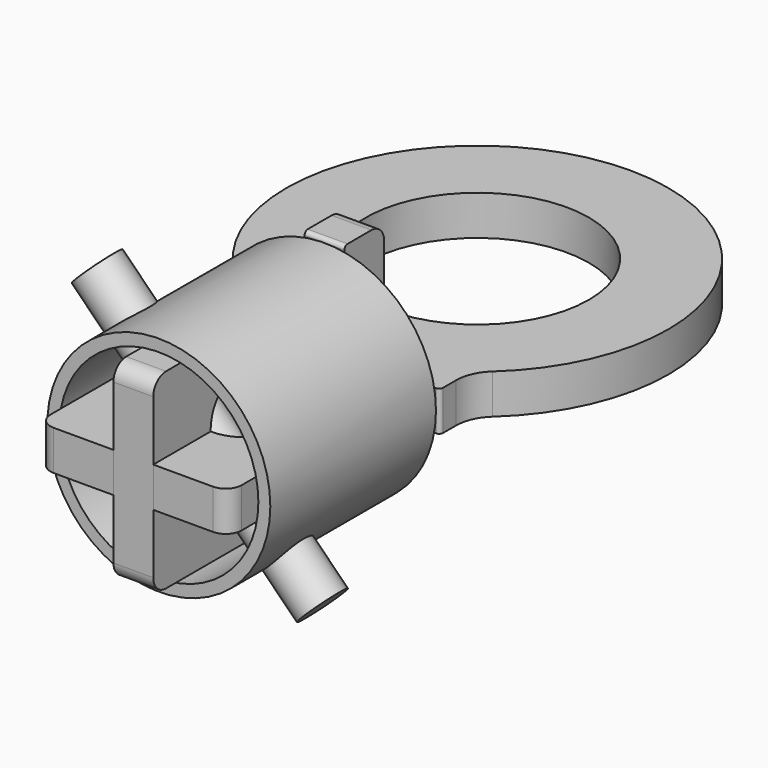
from build123d import *

# Parameters (mm, degrees)
F0_R      = 14
F1_DEPTH  = 2.5
F3_DEPTH  = 2.5
F6_START  = 24
F5_R      = 14
F5_R_2    = 12.5
F6_DEPTH  = 26
F8_R      = 3
F9_DEPTH  = 20
F13_DEPTH = 12.5
F16_DEPTH = 12.5
F17_R     = 2
F17_2_R   = 2
F18_R     = 2
F19_R     = 0.5
F19_2_R   = 0.5


with BuildPart() as f1:
    # F0 (on Top) → F1 (new body, symmetric)
    with BuildSketch(Plane.XY):
        with BuildLine():
            ThreePointArc((14.5, -21.4650879337), (14.9277825496, -19.4415199002), (16.1379310345, -17.7642107037))
            ThreePointArc((16.1379310345, -17.7642107037), (0, 24), (-16.1379310345, -17.7642107037))
            ThreePointArc((-16.1379310345, -17.7642107037), (-14.9277825496, -19.4415199002), (-14.5, -21.4650879337))
            Line((-14.5, -21.4650879337), (-14.5, -24))
            Line((-14.5, -24), (-12, -24))
            Line((-12, -24), (-12, -54))
            Line((-12, -54), (-2.5, -54))
            Line((-2.5, -54), (-2.5, -34))
            Line((-2.5, -34), (2.5, -34))
            Line((2.5, -34), (2.5, -54))
            Line((2.5, -54), (12, -54))
            Line((12, -54), (12, -24))
            Line((12, -24), (14.5, -24))
            Line((14.5, -24), (14.5, -21.4650879337))
        make_face()
        Circle(F0_R, mode=Mode.SUBTRACT)
    extrude(amount=F1_DEPTH, both=True)


with BuildPart() as f3:
    # F2 (on Right) → F3 (new body, symmetric)
    with BuildSketch(Plane.YZ):
        Polygon((-24, 14.5), (-24, 12), (-54, 12), (-54, -12), (-24, -12), (-24, -14.5), (-17.7642107037, -14.5), (-17.7642107037, 14.5), align=None)
    extrude(amount=F3_DEPTH, both=True)

    # F4: cut F1
    add(f1.part, mode=Mode.SUBTRACT)


with BuildPart() as f6:
    # F5 (on Front) → F6 (new body)
    with BuildSketch(Plane.XZ.offset(F6_START)):
        Circle(F5_R)
        Circle(F5_R_2, mode=Mode.SUBTRACT)
    extrude(amount=F6_DEPTH)


with BuildPart() as f9:
    # F8 (on face) → F9 (new body, symmetric)
    with BuildSketch(Plane(origin=(0, 0, 0), x_dir=(0, 1, 0), z_dir=(0.7071067812, 0, -0.7071067812))):
        with Locations((-42, 0)):
            Circle(F8_R)
    extrude(amount=F9_DEPTH, both=True)


with BuildPart() as f6_1:
    add(f6.part)

    # F10: cut F9
    add(f9.part, mode=Mode.SUBTRACT)


with BuildPart() as f3_1:
    add(f3.part)

    # F11: cut F9
    add(f9.part, mode=Mode.SUBTRACT)

    # F15 (on Right) → F16 (cut, symmetric)
    with BuildSketch(Plane.YZ):
        with BuildLine():
            Line((-45, 2.5), (-45, -2.5))
            add(Edge.make_bspline(
                [(-45, -2.5), (-45, -6.7426406871), (-42, -6.7426406871), (-39, -6.7426406871), (-39, -2.5)],
                knots=[1.5707963268, 1.5707963268, 1.5707963268, 3.1415926536, 3.1415926536, 4.7123889804, 4.7123889804, 4.7123889804], degree=2, weights=[1, 0.7071067812, 1, 0.7071067812, 1]))
            Line((-39, -2.5), (-39, 2.5))
            add(Edge.make_bspline(
                [(-39, 2.5), (-39, 6.7426406871), (-42, 6.7426406871), (-45, 6.7426406871), (-45, 2.5)],
                knots=[1.5707963268, 1.5707963268, 1.5707963268, 3.1415926536, 3.1415926536, 4.7123889804, 4.7123889804, 4.7123889804], degree=2, weights=[1, 0.7071067812, 1, 0.7071067812, 1]))
        make_face()
    extrude(amount=F16_DEPTH, both=True, mode=Mode.SUBTRACT)

    # F17#2
    f17_2_edges = [f3_1.edges().sort_by_distance(p)[0] for p in [
        (0, -54, 12),
        (0, -54, -12),
    ]]
    fillet(f17_2_edges, radius=F17_2_R)

    # F18
    f18_edges = [f3_1.edges().sort_by_distance(p)[0] for p in [
        (0, -17.764211, -14.5),
        (0, -17.764211, 14.5),
    ]]
    fillet(f18_edges, radius=F18_R)

    # F19#2
    f19_2_edges = [f3_1.edges().sort_by_distance(p)[0] for p in [
        (0, -24, 14.5),
        (0, -24, -14.5),
    ]]
    fillet(f19_2_edges, radius=F19_2_R)


with BuildPart() as f1_1:
    add(f1.part)

    # F11: cut F9
    add(f9.part, mode=Mode.SUBTRACT)


with BuildPart() as f13:
    # F12 (on Top) → F13 (new body, symmetric)
    with BuildSketch(Plane.XY):
        with BuildLine():
            Line((2.5, -39), (-2.5, -39))
            add(Edge.make_bspline(
                [(-2.5, -39), (-6.7426406871, -39), (-6.7426406871, -42), (-6.7426406871, -45), (-2.5, -45)],
                knots=[4.7123889804, 4.7123889804, 4.7123889804, 6.2831853072, 6.2831853072, 7.853981634, 7.853981634, 7.853981634], degree=2, weights=[1, 0.7071067812, 1, 0.7071067812, 1]))
            Line((-2.5, -45), (2.5, -45))
            add(Edge.make_bspline(
                [(2.5, -45), (6.7426406871, -45), (6.7426406871, -42), (6.7426406871, -39), (2.5, -39)],
                knots=[4.7123889804, 4.7123889804, 4.7123889804, 6.2831853072, 6.2831853072, 7.853981634, 7.853981634, 7.853981634], degree=2, weights=[1, 0.7071067812, 1, 0.7071067812, 1]))
        make_face()
    extrude(amount=F13_DEPTH, both=True)


with BuildPart() as f1_2:
    add(f1_1.part)

    # F14: cut F13
    add(f13.part, mode=Mode.SUBTRACT)

    # F17
    f17_edges = [f1_2.edges().sort_by_distance(p)[0] for p in [
        (12, -54, 0),
        (-12, -54, 0),
    ]]
    fillet(f17_edges, radius=F17_R)

    # F19
    f19_edges = [f1_2.edges().sort_by_distance(p)[0] for p in [
        (14.5, -24, 0),
        (-14.5, -24, 0),
    ]]
    fillet(f19_edges, radius=F19_R)


solid = Compound([f9.part, f6_1.part, f3_1.part, f1_2.part])
